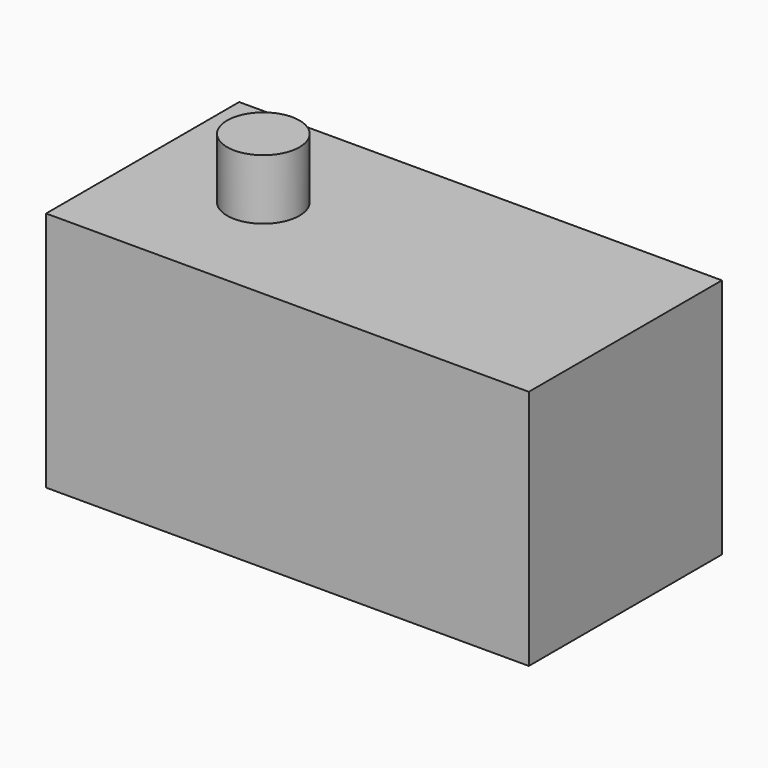
from build123d import *

# Parameters (mm, degrees)
F0_W     = 120
F0_H     = 60
F1_DEPTH = 30
F2_R     = 9
F3_DEPTH = 15
F4_DEPTH = 15
F6_DEPTH = 25


# Not quite as in the source:
# - the program builds the solid bodies; features that only make, move or delete a surface that nothing else refers to are left out


with BuildPart() as f1:
    # F0 (on Front) → F1 (new body, symmetric)
    with BuildSketch(Plane.XZ):
        with Locations((60, 30)):
            Rectangle(F0_W, F0_H)
    extrude(amount=F1_DEPTH, both=True)

    # F2 (on face) → F3 (join)
    with BuildSketch(Plane.XY.offset(60)):
        with Locations((30, 0)):
            Circle(F2_R)
    extrude(amount=F3_DEPTH)

    # F2 (on face) → F4 (join)
    with BuildSketch(Plane.XY.offset(60)):
        with Locations((30, 0)):
            Circle(F2_R)
        with Locations((60, 0)):
            Circle(F2_R)
        with Locations((90, 0)):
            Circle(F2_R)
    extrude(amount=-F4_DEPTH)

    # F0 (on Front) → F6 (join)
    with BuildSketch(Plane.XZ):
        with Locations((60, 30)):
            Rectangle(F0_W, F0_H)
    extrude(amount=F6_DEPTH)


solid = f1.part
